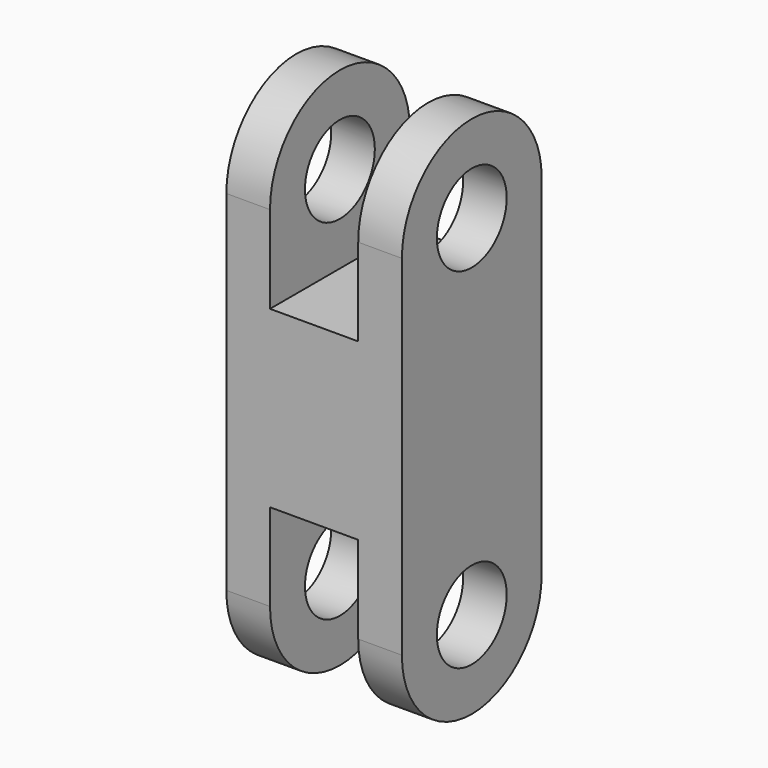
from build123d import *

# Parameters (mm, degrees)
F0_W     = 40
F0_H     = 80
F1_DEPTH = 20.1
F3_R     = 10
F4_DEPTH = 10
F6_W     = 20.2
F6_H     = 40
F7_DEPTH = 40
F8_R     = 10
F9_DEPTH = 40.2
F10_R    = 19.99999


# Not quite as in the source:
# - a fillet or chamfer is up to 0.001 mm smaller than in the source, because OpenCascade refuses the exact size


with BuildPart() as f1:
    # F0 (on Right) → F1 (new body)
    with BuildSketch(Plane.YZ):
        Rectangle(F0_W, F0_H)
    extrude(amount=F1_DEPTH)

    # F3 (on face) → F4 (join)
    with BuildSketch(Plane.YZ.offset(20.1)):
        with BuildLine():
            Line((-20, 60), (-20, 40))
            Line((-20, 40), (20, 40))
            Line((20, 40), (20, 60))
            ThreePointArc((20, 60), (0, 80), (-20, 60))
        make_face()
        with Locations((0, 60)):
            Circle(F3_R, mode=Mode.SUBTRACT)
    extrude(amount=-F4_DEPTH)

    # F5: F1 across plane


with BuildPart() as f1_1:
    add(f1.part)
    add(f1.part.mirror(Plane.YZ))

    # F6 (on face) → F7 (cut, through all)
    with BuildSketch(Plane.XZ.offset(20)):
        with Locations((0, -20)):
            Rectangle(F6_W, F6_H)
    extrude(amount=-F7_DEPTH, mode=Mode.SUBTRACT)

    # F8 (on face) → F9 (cut, through all)
    with BuildSketch(Plane.YZ.offset(20.1)):
        with Locations((0, -20)):
            Circle(F8_R)
    extrude(amount=-F9_DEPTH, mode=Mode.SUBTRACT)

    # F10 (radius 20 in the source; OpenCascade refuses exactly that, so slightly less here)
    f10_edges = [f1_1.edges().sort_by_distance(p)[0] for p in [
        (15.1, -20, -40),
        (-15.1, -20, -40),
        (-15.1, 20, -40),
        (15.1, 20, -40),
    ]]
    fillet(f10_edges, radius=F10_R)


solid = f1_1.part
